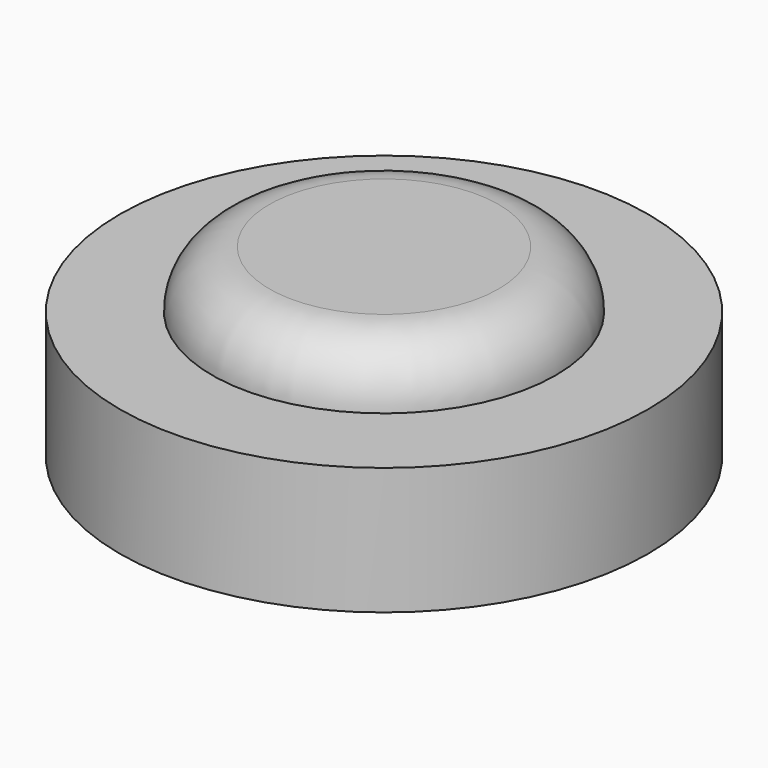
from build123d import *

# Parameters (mm, degrees)
F0_R     = 15
F0_R_2   = 14
F1_DEPTH = 5
F2_DEPTH = 10
F0_R_3   = 23.05
F3_DEPTH = 11.1
F4_R     = 4.99999


# Not quite as in the source:
# - a fillet or chamfer is up to 0.001 mm smaller than in the source, because OpenCascade refuses the exact size


with BuildPart() as f1:
    # F0 (on Top) → F1 (new body)
    with BuildSketch(Plane.XY):
        Circle(F0_R)
        Circle(F0_R_2, mode=Mode.SUBTRACT)
        Circle(F0_R_2)
    extrude(amount=F1_DEPTH)

    # F4 (radius 5 in the source; OpenCascade refuses exactly that, so slightly less here)
    f4_edges = [f1.edges().sort_by_distance(p)[0] for p in [
        (-15, 0, 5),
    ]]
    fillet(f4_edges, radius=F4_R)


with BuildPart() as f2:
    # F0 (on Top) → F2 (new body)
    with BuildSketch(Plane.XY):
        Circle(F0_R_2)
    extrude(amount=-F2_DEPTH)


with BuildPart() as f3:
    # F0 (on Top) → F3 (new body)
    with BuildSketch(Plane.XY):
        Circle(F0_R_3)
        Circle(F0_R, mode=Mode.SUBTRACT)
        Circle(F0_R)
        Circle(F0_R_2, mode=Mode.SUBTRACT)
    extrude(amount=-F3_DEPTH)


solid = Compound([f1.part, f2.part, f3.part])
